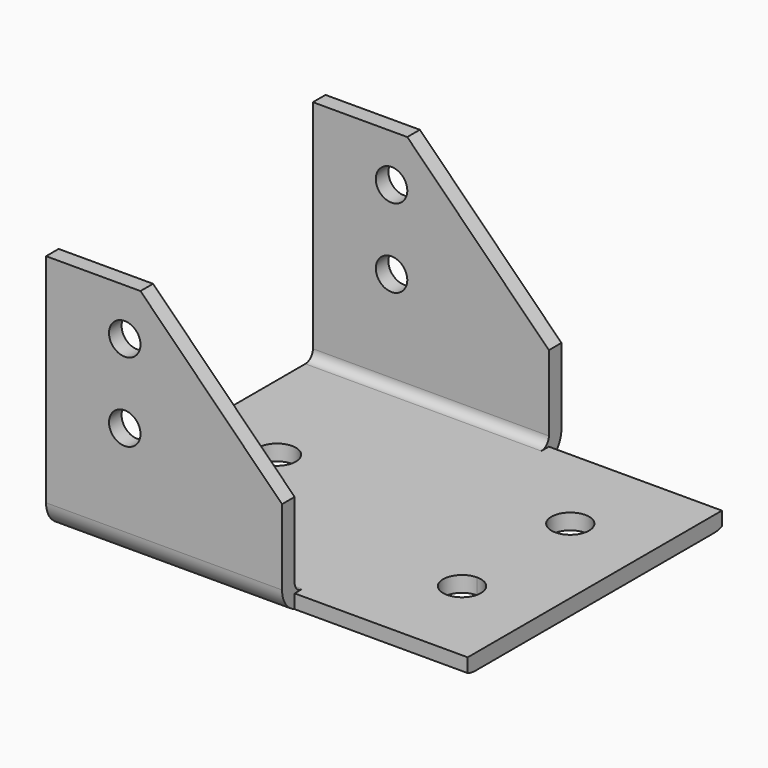
from build123d import *

# Parameters (mm, degrees)
F1_DEPTH = 5
F0_W     = 75
F0_H     = 5
F2_DEPTH = 77
F3_SIZE  = 45
F4_SIZE  = 45
F5_R     = 3
F6_R     = 8
F8_D     = 10
F9_D     = 10


with BuildPart() as f1:
    # F0 (on Top) → F1 (new body)
    with BuildSketch(Plane.XY):
        Polygon((30, 23.6378825456), (55, 23.6378825456), (55, 124.6378825456), (0, 124.6378825456), (-75, 124.6378825456), (-75, 79.1378825456), (-75, 23.6378825456), (0, 23.6378825456), align=None)
        with BuildLine():
            ThreePointArc((36, 52.6378825456), (34.2426406871, 48.3952418585), (30, 46.6378825456))
            ThreePointArc((30, 46.6378825456), (24, 52.6378825456), (30, 58.6378825456))
            ThreePointArc((30, 58.6378825456), (34.2426406871, 56.8805232327), (36, 52.6378825456))
        make_face(mode=Mode.SUBTRACT)
        with BuildLine():
            ThreePointArc((-44, 79.1378825456), (-50, 73.1378825456), (-56, 79.1378825456))
            ThreePointArc((-56, 79.1378825456), (-50, 85.1378825456), (-44, 79.1378825456))
        make_face(mode=Mode.SUBTRACT)
        with BuildLine():
            ThreePointArc((36, 95.6378825456), (34.2426406871, 91.3952418585), (30, 89.6378825456))
            ThreePointArc((30, 89.6378825456), (25.7573593129, 99.8805232327), (36, 95.6378825456))
        make_face(mode=Mode.SUBTRACT)
    extrude(amount=F1_DEPTH)

    # F0 (on Top) → F2 (join)
    with BuildSketch(Plane.XY):
        with Locations((-37.5, 127.1378825456)):
            Rectangle(F0_W, F0_H)
        with Locations((-37.5, 21.1378825456)):
            Rectangle(F0_W, F0_H)
    extrude(amount=F2_DEPTH)

    # F3
    f3_edges = [f1.edges().sort_by_distance(p)[0] for p in [
        (0, 127.137883, 77),
    ]]
    chamfer(f3_edges, length=F3_SIZE)

    # F4
    f4_edges = [f1.edges().sort_by_distance(p)[0] for p in [
        (0, 21.137883, 77),
    ]]
    chamfer(f4_edges, length=F4_SIZE)

    # F5
    f5_edges = [f1.edges().sort_by_distance(p)[0] for p in [
        (-37.5, 124.637883, 5),
        (-37.5, 23.637883, 5),
    ]]
    fillet(f5_edges, radius=F5_R)

    # F6
    f6_edges = [f1.edges().sort_by_distance(p)[0] for p in [
        (-37.5, 18.637883, 0),
        (-37.5, 129.637883, 0),
    ]]
    fillet(f6_edges, radius=F6_R)

    # F8 (through all)
    with Locations(Plane.XZ.offset(-18.6378825456)):
        with Locations((-50, 37)):
            Hole(F8_D / 2)

    # F9 (through all)
    with Locations(Plane.XZ.offset(-18.6378825456)):
        with Locations((-50, 62)):
            Hole(F9_D / 2)


solid = f1.part
